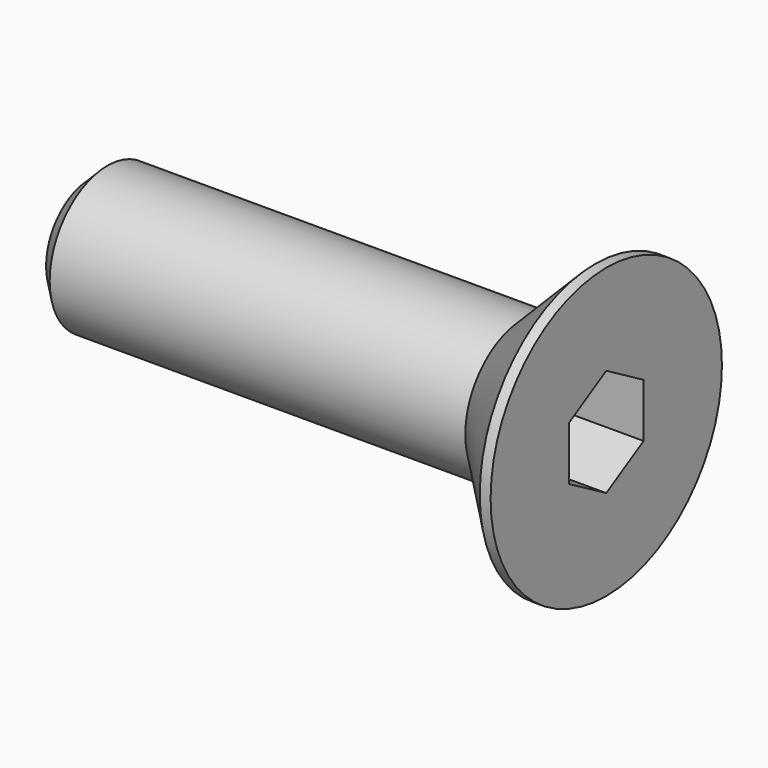
from build123d import *

# Parameters (mm, degrees)
F0_R     = 4
F1_DEPTH = 2.3
F2_R     = 2
F3_DEPTH = 12
F4_SIZE  = 0.5
F5_SIZE2 = 1.99999
F5_SIZE  = 1.99999
F7_DEPTH = 2


# Not quite as in the source:
# - a fillet or chamfer is up to 0.001 mm smaller than in the source, because OpenCascade refuses the exact size


with BuildPart() as f1:
    # F0 (on Right) → F1 (new body)
    with BuildSketch(Plane.YZ):
        Circle(F0_R)
    extrude(amount=-F1_DEPTH)

    # F2 (on face) → F3 (join)
    with BuildSketch(Plane(origin=(-2.3, 0, 0), x_dir=(0, -1, 0), z_dir=(-1, 0, 0))):
        Circle(F2_R)
    extrude(amount=F3_DEPTH)

    # F4
    f4_edges = [f1.edges().sort_by_distance(p)[0] for p in [
        (-14.3, 2, 0),
    ]]
    chamfer(f4_edges, length=F4_SIZE)

    # F5 (size 2 and 2 in the source; OpenCascade refuses exactly that, so slightly less here)
    f5_edges = [f1.edges().sort_by_distance(p)[0] for p in [
        (-2.3, -4, 0),
    ]]
    chamfer(f5_edges, length=F5_SIZE, length2=F5_SIZE2)

    # F6 (on face) → F7 (cut)
    with BuildSketch(Plane.YZ):
        Polygon((0, -1.4895636945), (1.29, -0.7447818473), (1.29, 0.7447818473), (0, 1.4895636945), (-1.29, 0.7447818473), (-1.29, -0.7447818473), align=None)
    extrude(amount=-F7_DEPTH, mode=Mode.SUBTRACT)


solid = f1.part
